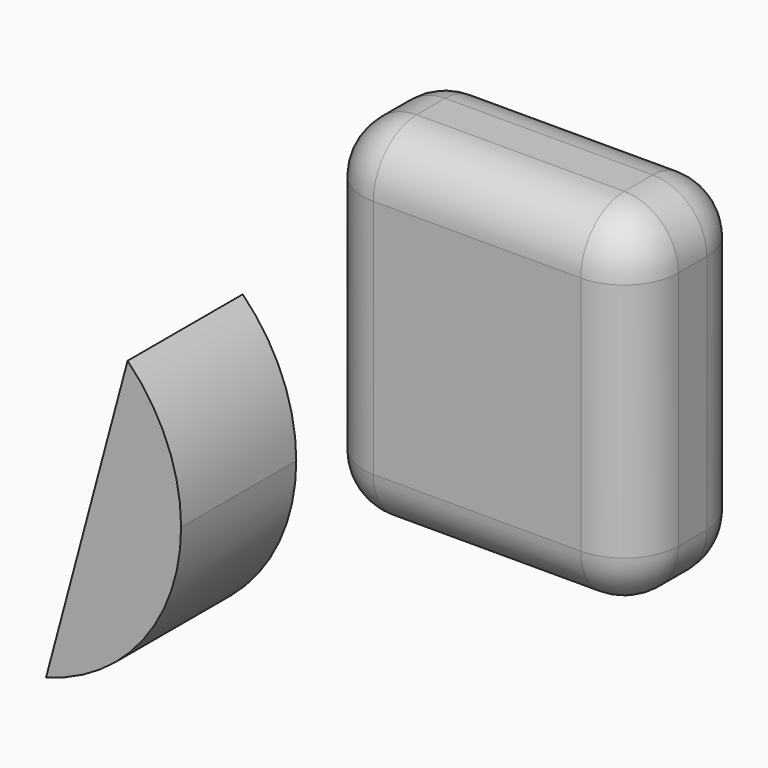
from build123d import *

# Parameters (mm, degrees)
F2_DEPTH = 25
F3_W     = 54.8490260262
F3_H     = 60.5938415974
F4_DEPTH = 25
F5_R     = 9.4154328933


# Not quite as in the source:
# - the program builds the solid bodies; features that only make, move or delete a surface that nothing else refers to are left out


with BuildPart() as f2:
    # F0 (on Front) → F2 (new body)
    with BuildSketch(Plane.XZ):
        with BuildLine():
            ThreePointArc((-99.0687261738, -24.5411251405), (-82.1541433894, -13.2232410682), (-75.616435726, 6.0499524698))
            ThreePointArc((-75.616435726, 6.0499524698), (-78.0330079972, 18.1851301237), (-84.9140211289, 28.4688073121))
            Line((-84.9140211289, 28.4688073121), (-99.0687261738, -24.5411251405))
        make_face()
    extrude(amount=F2_DEPTH)


with BuildPart() as f4:
    # F3 (on Front) → F4 (new body)
    with BuildSketch(Plane.XZ):
        with Locations((-24.2105474463, 45.8376193419)):
            Rectangle(F3_W, F3_H)
    extrude(amount=F4_DEPTH)

    # F5
    f5_edges = [f4.edges().sort_by_distance(p)[0] for p in [
        (-51.63506, -25, 45.837619),
        (-24.210547, -25, 15.540699),
        (-24.210547, 0, 15.540699),
        (3.213966, -12.5, 15.540699),
        (-51.63506, -12.5, 15.540699),
        (-51.63506, -12.5, 76.13454),
        (3.213966, -25, 45.837619),
        (-51.63506, 0, 45.837619),
        (-24.210547, -25, 76.13454),
        (-24.210547, 0, 76.13454),
        (3.213966, 0, 45.837619),
        (3.213966, -12.5, 76.13454),
    ]]
    fillet(f5_edges, radius=F5_R)


solid = Compound([f2.part, f4.part])
